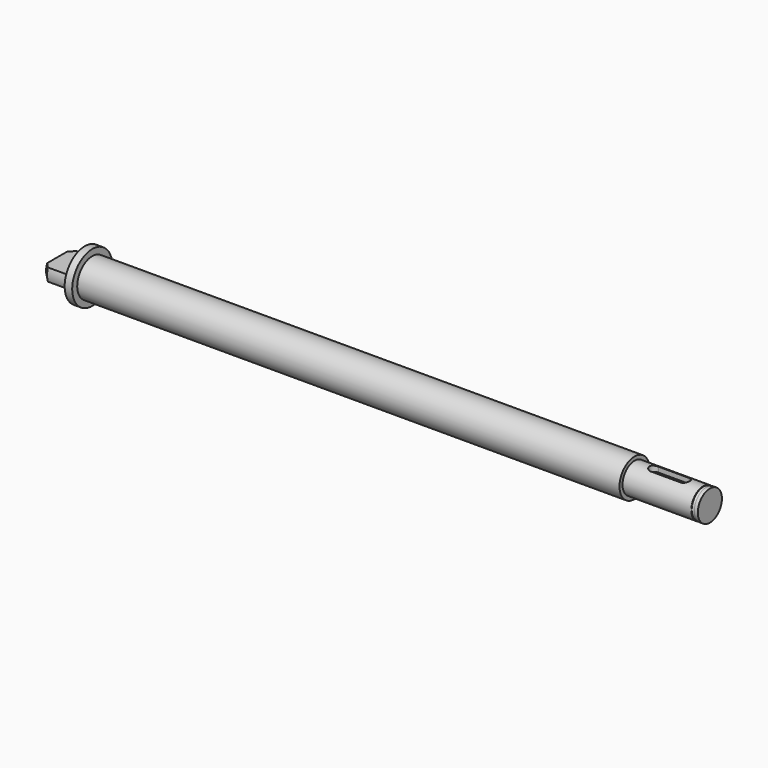
from build123d import *

# Parameters (mm, degrees)
F2_SIZE  = 1
F4_DEPTH = 5.5
F7_DEPTH = 1.2


with BuildPart() as f1:
    # F0 (on Front) → F1 (revolve)
    with BuildSketch(Plane.XZ):
        Polygon((0, 3.75), (0, 0), (130, 0), (130, 3), (129.3, 3), (129.3, 2.9), (128.7, 2.9), (128.7, 3), (115, 3), (115, 3.75), (7, 3.75), (7, 5), (5.5, 5), (5.5, 3.75), align=None)
    revolve(axis=Axis((81.1427264533, 0, 0), (1, 0, 0)))

    # F2
    f2_edges = [f1.edges().sort_by_distance(p)[0] for p in [
        (0, 0, -3.75),
    ]]
    chamfer(f2_edges, length=F2_SIZE)

    # F3 (on face) → F4 (cut, through all)
    with BuildSketch(Plane(origin=(0, 0, 0), x_dir=(0, -1, 0), z_dir=(-1, 0, 0))):
        with BuildLine():
            Line((2.4494897428, 1.25), (3.5355339059, 1.25))
            ThreePointArc((3.5355339059, 1.25), (0, 3.75), (-3.5355339059, 1.25))
            Line((-3.5355339059, 1.25), (-2.4494897428, 1.25))
            ThreePointArc((-2.4494897428, 1.25), (0, 2.75), (2.4494897428, 1.25))
        make_face()
        with BuildLine():
            ThreePointArc((-3.5355339059, -1.25), (0, -3.75), (3.5355339059, -1.25))
            Line((3.5355339059, -1.25), (2.4494897428, -1.25))
            ThreePointArc((2.4494897428, -1.25), (0, -2.75), (-2.4494897428, -1.25))
            Line((-2.4494897428, -1.25), (-3.5355339059, -1.25))
        make_face()
        with BuildLine():
            Line((-2.4494897428, 1.25), (2.4494897428, 1.25))
            ThreePointArc((2.4494897428, 1.25), (0, 2.75), (-2.4494897428, 1.25))
        make_face()
        with BuildLine():
            ThreePointArc((-2.4494897428, -1.25), (0, -2.75), (2.4494897428, -1.25))
            Line((2.4494897428, -1.25), (-2.4494897428, -1.25))
        make_face()
    extrude(amount=-F4_DEPTH, mode=Mode.SUBTRACT)

    # F6 (on offset) → F7 (cut, through all)
    with BuildSketch(Plane.XY.offset(1.8)):
        with BuildLine():
            ThreePointArc((125, -1), (126, 0), (125, 1))
            Line((125, 1), (119, 1))
            ThreePointArc((119, 1), (118, 0), (119, -1))
            Line((119, -1), (125, -1))
        make_face()
    extrude(amount=F7_DEPTH, mode=Mode.SUBTRACT)


solid = f1.part
